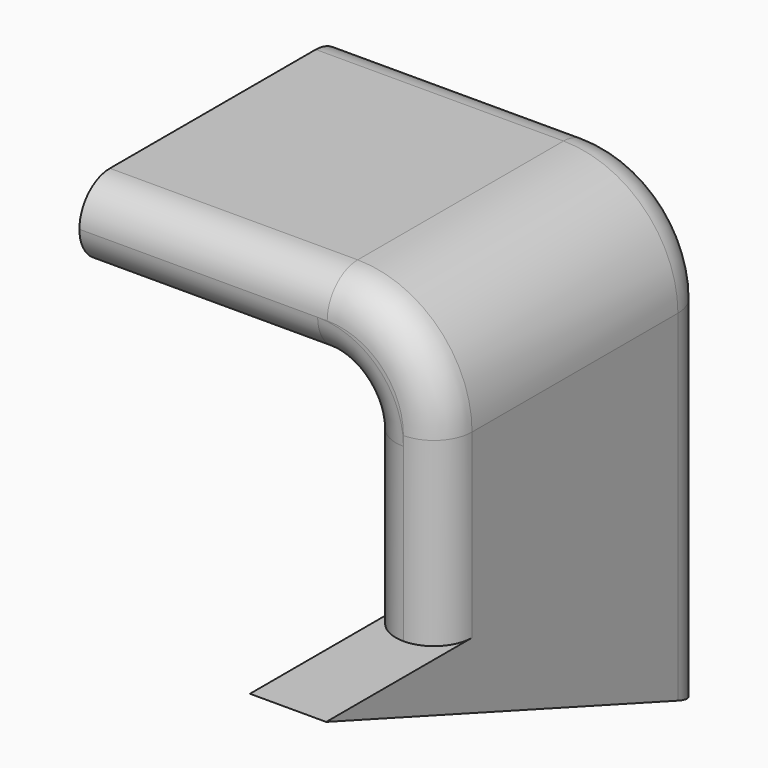
from build123d import *

# Parameters (mm, degrees)
F1_DEPTH = 35
F3_DEPTH = 8
F4_R     = 5
F5_R     = 12
F6_R     = 3.99999
F7_R     = 3.99999


# Not quite as in the source:
# - a fillet or chamfer is up to 0.001 mm smaller than in the source, because OpenCascade refuses the exact size


with BuildPart() as f1:
    # F0 (on Front) → F1 (new body)
    with BuildSketch(Plane.XZ):
        Polygon((-30, 31), (-30, 23), (0, 23), (0, 0), (8, 0), (8, 31), align=None)
    extrude(amount=F1_DEPTH)

    # F2 (on Right) → F3 (join)
    with BuildSketch(Plane.YZ):
        Polygon((0, 0), (-50.1344501972, 0), (0, -18.2474475831), align=None)
    extrude(amount=F3_DEPTH)

    # F4
    f4_edges = [f1.edges().sort_by_distance(p)[0] for p in [
        (0, -17.5, 23),
    ]]
    fillet(f4_edges, radius=F4_R)

    # F5
    f5_edges = [f1.edges().sort_by_distance(p)[0] for p in [
        (8, -17.5, 31),
    ]]
    fillet(f5_edges, radius=F5_R)

    # F6 (radius 4 in the source; OpenCascade refuses exactly that, so slightly less here)
    f6_edges = [f1.edges().sort_by_distance(p)[0] for p in [
        (-17, -35, 31),
        (-17.5, -35, 23),
        (4.485281, -35, 27.485281),
        (-1.464466, -35, 21.535534),
        (0, -35, 9),
        (8, -35, 9.5),
    ]]
    fillet(f6_edges, radius=F6_R)

    # F7 (radius 4 in the source; OpenCascade refuses exactly that, so slightly less here)
    f7_edges = [f1.edges().sort_by_distance(p)[0] for p in [
        (-17, 0, 31),
        (-17.5, 0, 23),
        (0, 0, -0.123724),
        (8, 0, 0.376276),
        (4.485281, 0, 27.485281),
        (-1.464466, 0, 21.535534),
    ]]
    fillet(f7_edges, radius=F7_R)


solid = f1.part
